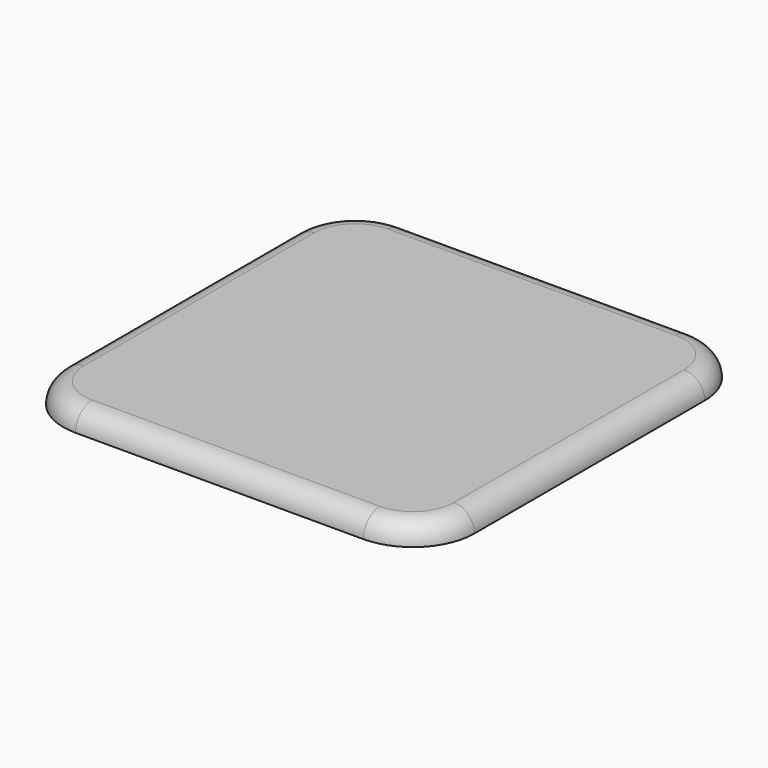
from build123d import *

# Parameters (mm, degrees)
F1_DEPTH = 5
F2_R     = 4.99999


# Not quite as in the source:
# - a fillet or chamfer is up to 0.001 mm smaller than in the source, because OpenCascade refuses the exact size


with BuildPart() as f1:
    # F0 (on Top) → F1 (new body)
    with BuildSketch(Plane.XY):
        with BuildLine():
            Line((35, 50), (-35, 50))
            ThreePointArc((-35, 50), (-45.6066017178, 45.6066017178), (-50, 35))
            Line((-50, 35), (-50, -35))
            ThreePointArc((-50, -35), (-45.6066017178, -45.6066017178), (-35, -50))
            Line((-35, -50), (35, -50))
            ThreePointArc((35, -50), (45.6066017178, -45.6066017178), (50, -35))
            Line((50, -35), (50, 35))
            ThreePointArc((50, 35), (45.6066017178, 45.6066017178), (35, 50))
        make_face()
    extrude(amount=F1_DEPTH)

    # F2 (radius 5 in the source; OpenCascade refuses exactly that, so slightly less here)
    f2_edges = [f1.edges().sort_by_distance(p)[0] for p in [
        (0, 50, 5),
        (-45.606602, 45.606602, 5),
        (-50, 0, 5),
        (-45.606602, -45.606602, 5),
        (0, -50, 5),
        (45.606602, -45.606602, 5),
        (50, 0, 5),
        (45.606602, 45.606602, 5),
    ]]
    fillet(f2_edges, radius=F2_R)


solid = f1.part
